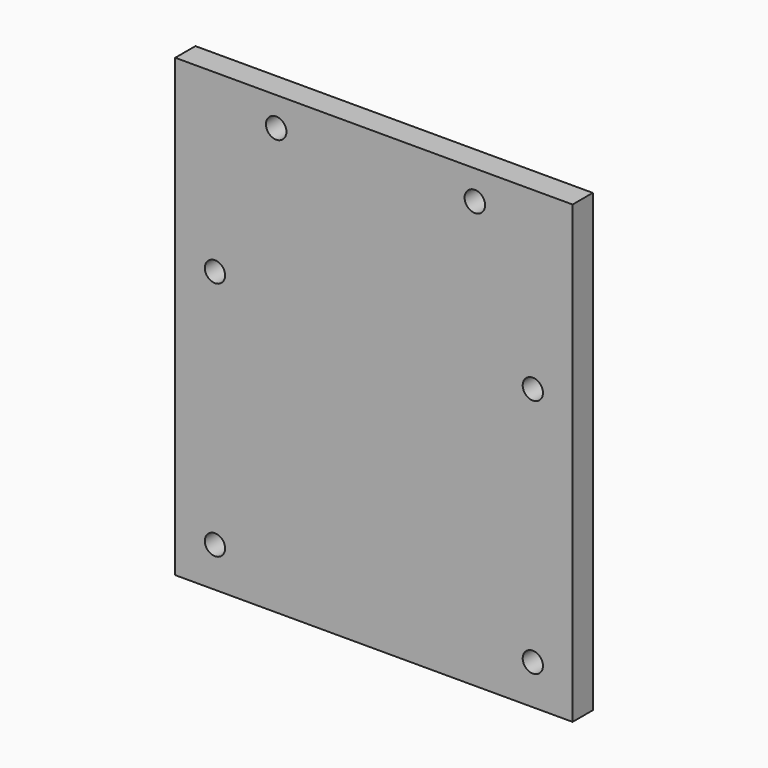
from build123d import *

# Parameters (mm, degrees)
F0_R     = 2.55
F0_R_2   = 2.58
F1_DEPTH = 6.35


# Not quite as in the source:
# - a feature names something its author has since deleted; it is built from what else it names


with BuildPart() as f1:
    # F0 (on Front) → F1 (new body)
    with BuildSketch(Plane.XZ):
        Polygon((-50, -50), (50, -50), (50, 50), (50, 64.6395087242), (-50, 64.6395087242), (-50, 50), align=None)
        with Locations((-40, -40)):
            Circle(F0_R, mode=Mode.SUBTRACT)
        with Locations((40, -40)):
            Circle(F0_R, mode=Mode.SUBTRACT)
        with Locations((-40, 20.49)):
            Circle(F0_R, mode=Mode.SUBTRACT)
        with Locations((-24.5967630297, 57.3197543621)):
            Circle(F0_R_2, mode=Mode.SUBTRACT)
        with Locations((40, 20.49)):
            Circle(F0_R, mode=Mode.SUBTRACT)
        with Locations((25.4032369703, 57.3197543621)):
            Circle(F0_R_2, mode=Mode.SUBTRACT)
    extrude(amount=F1_DEPTH)


solid = f1.part
